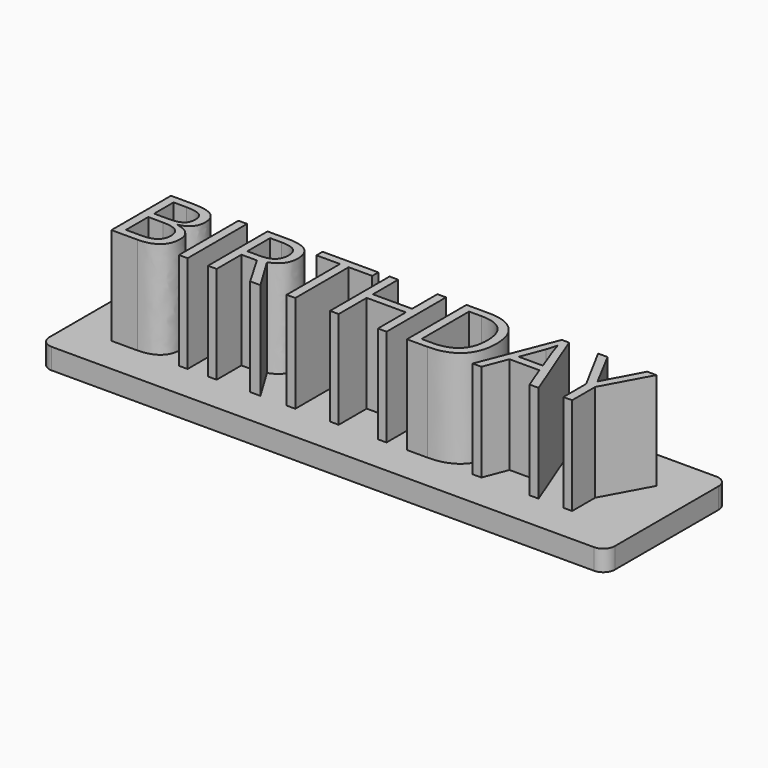
from build123d import *

# Parameters (mm, degrees)
F1_DEPTH     = 1.8
F2_TEXT_SIZE = 9.0277777778
F3_DEPTH     = 8.45


# Not quite as in the source:
# - Text() gives the source's letters only with a copy of the font that has no kerning and outlines rounded to 1/6400 em; it was checked with that copy


with BuildPart() as f1:
    # F0 (on Top) → F1 (new body)
    with BuildSketch(Plane.XY):
        with BuildLine():
            ThreePointArc((24.5, 5.625), (24.2071067812, 6.3321067812), (23.5, 6.625))
            Line((23.5, 6.625), (-23.5, 6.625))
            ThreePointArc((-23.5, 6.625), (-24.2071067812, 6.3321067812), (-24.5, 5.625))
            Line((-24.5, 5.625), (-24.5, -5.625))
            ThreePointArc((-24.5, -5.625), (-24.2071067812, -6.3321067812), (-23.5, -6.625))
            Line((-23.5, -6.625), (23.5, -6.625))
            ThreePointArc((23.5, -6.625), (24.2071067812, -6.3321067812), (24.5, -5.625))
            Line((24.5, -5.625), (24.5, 5.625))
        make_face()
    extrude(amount=F1_DEPTH)

    # F2 (on face) → F3 (join)
    with BuildSketch(Plane.XY.offset(1.8)):
        with Locations((-21.7689344618, -3.4158185796)):
            Text('BIRTHDAY', F2_TEXT_SIZE, font='Open Sans', text_align=(TextAlign.LEFT, TextAlign.BOTTOM))
    extrude(amount=F3_DEPTH)


solid = f1.part
